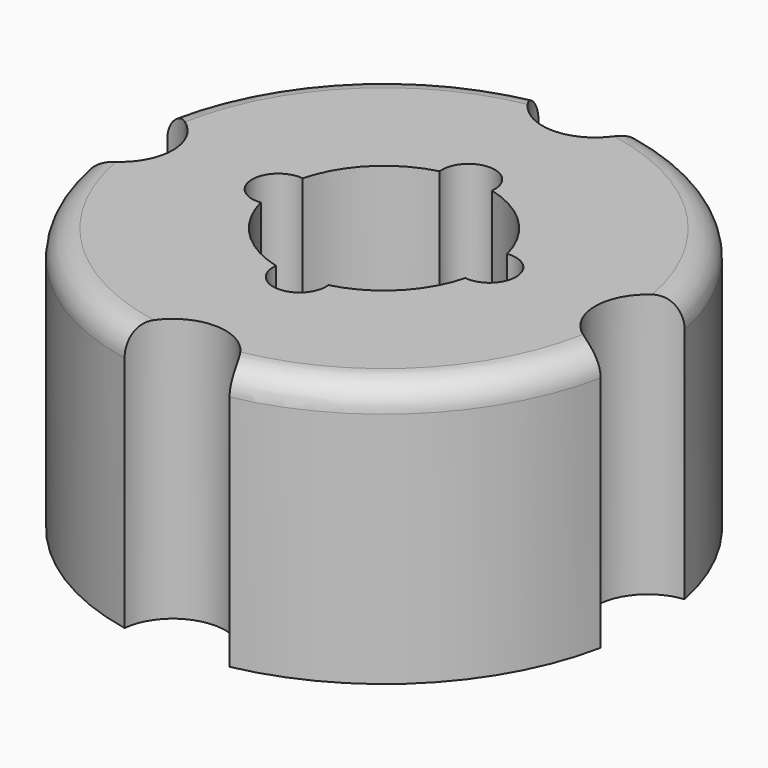
from build123d import *

# Parameters (mm, degrees)
F1_DEPTH = 50
F5_R     = 5


# Not quite as in the source:
# - the program builds the solid bodies; features that only make, move or delete a surface that nothing else refers to are left out


with BuildPart() as f1:
    # F0 (on Top) → F1 (new body)
    with BuildSketch(Plane.XY):
        with BuildLine():
            ThreePointArc((9.9498743711, 49), (0, 40), (-9.9498743711, 49))
            ThreePointArc((-9.9498743711, 49), (-35.3553390593, 35.3553390593), (-49, 9.9498743711))
            ThreePointArc((-49, 9.9498743711), (-40, 0), (-49, -9.9498743711))
            ThreePointArc((-49, -9.9498743711), (-35.3553390593, -35.3553390593), (-9.9498743711, -49))
            ThreePointArc((-9.9498743711, -49), (0, -40), (9.9498743711, -49))
            ThreePointArc((9.9498743711, -49), (35.3553390593, -35.3553390593), (49, -9.9498743711))
            ThreePointArc((49, -9.9498743711), (40, 0), (49, 9.9498743711))
            ThreePointArc((49, 9.9498743711), (35.3553390593, 35.3553390593), (9.9498743711, 49))
        make_face()
        with BuildLine():
            ThreePointArc((-4.9607837082, -19.375), (-14.1421356237, -14.1421356237), (-19.375, -4.9607837082))
            ThreePointArc((-19.375, -4.9607837082), (-25, 0), (-19.375, 4.9607837082))
            ThreePointArc((-19.375, 4.9607837082), (-14.1421356237, 14.1421356237), (-4.9607837082, 19.375))
            ThreePointArc((-4.9607837082, 19.375), (0, 25), (4.9607837082, 19.375))
            ThreePointArc((4.9607837082, 19.375), (14.1421356237, 14.1421356237), (19.375, 4.9607837082))
            ThreePointArc((19.375, 4.9607837082), (25, 0), (19.375, -4.9607837082))
            ThreePointArc((19.375, -4.9607837082), (14.1421356237, -14.1421356237), (4.9607837082, -19.375))
            ThreePointArc((4.9607837082, -19.375), (0, -25), (-4.9607837082, -19.375))
        make_face(mode=Mode.SUBTRACT)
    extrude(amount=F1_DEPTH)

    # F5
    f5_edges = [f1.edges().sort_by_distance(p)[0] for p in [
        (35.355339, -35.355339, 50),
        (35.355339, 35.355339, 50),
        (-35.355339, -35.355339, 50),
        (-35.355339, 35.355339, 50),
    ]]
    fillet(f5_edges, radius=F5_R)


solid = f1.part
